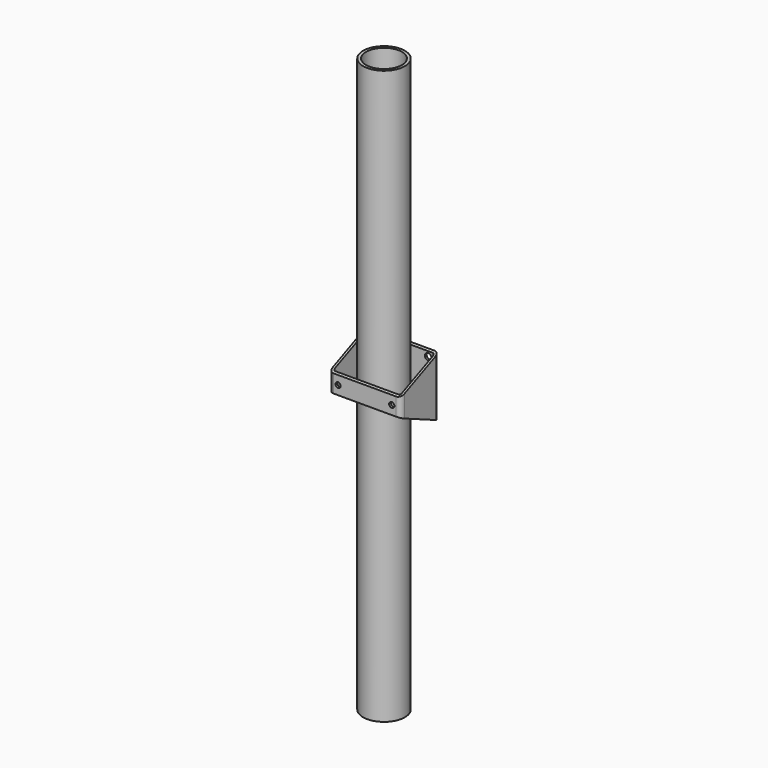
from build123d import *

# Parameters (mm, degrees)
F5_REACH        = 246.7313465507
F7_R            = 44.45
F7_R_2          = 38.1000004709
F8_DEPTH        = 609.6
F8_DEPTH_BACK   = 609.6
F10_D           = 14.3002
F11_D           = 11.1125
F11_CSINK_D     = 19.05
F11_CSINK_ANGLE = 90


with BuildPart() as f5:
    f5_end = Plane(origin=(0, 50.6421849132, 63.5), x_dir=(0, 0.9155220939, 0.4022676914), z_dir=(0, -0.4022676914, 0.9155220939))
    # F0 (on Top) → F5 (new body, up to a plane its end follows)
    with BuildSketch(Plane.XY):
        with BuildLine():
            ThreePointArc((76.2, 41.275), (73.4101920908, 48.0101920908), (66.675, 50.8))
            Line((66.675, 50.8), (-66.675, 50.8))
            ThreePointArc((-66.675, 50.8), (-73.4101920908, 48.0101920908), (-76.2, 41.275))
            Line((-76.2, 41.275), (-76.2, -41.275))
            ThreePointArc((-76.2, -41.275), (-73.4101920908, -48.0101920908), (-66.675, -50.8))
            Line((-66.675, -50.8), (66.675, -50.8))
            ThreePointArc((66.675, -50.8), (73.4101920908, -48.0101920908), (76.2, -41.275))
            Line((76.2, -41.275), (76.2, 41.275))
        make_face()
        with BuildLine():
            ThreePointArc((66.675, 46.0375), (70.0425960454, 44.6425960454), (71.4375, 41.275))
            Line((71.4375, 41.275), (71.4375, -41.275))
            ThreePointArc((71.4375, -41.275), (70.0425960454, -44.6425960454), (66.675, -46.0375))
            Line((66.675, -46.0375), (-66.675, -46.0375))
            ThreePointArc((-66.675, -46.0375), (-70.0425960454, -44.6425960454), (-71.4375, -41.275))
            Line((-71.4375, -41.275), (-71.4375, 41.275))
            ThreePointArc((-71.4375, 41.275), (-70.0425960454, 44.6425960454), (-66.675, 46.0375))
            Line((-66.675, 46.0375), (66.675, 46.0375))
        make_face(mode=Mode.SUBTRACT)
    f5_long = extrude(amount=F5_REACH, mode=Mode.PRIVATE)
    add(split(f5_long, bisect_by=f5_end, keep=Keep.BOTTOM, mode=Mode.PRIVATE))

    # F6: F5 across plane


with BuildPart() as f5_1:
    add(f5.part)
    add(f5.part.mirror(Plane.XY))

    # F10 (through all)
    with Locations(Plane(origin=(0, 50.8, 0), x_dir=(-1, 0, 0), z_dir=(0, 1, 0))):
        with Locations((-57.15, 50.8), (57.15, 50.8), (57.15, -50.8), (-57.15, -50.8)):
            Hole(F10_D / 2)

    # F11 (through all)
    with Locations(Plane(origin=(0, 50.8, 0), x_dir=(-1, 0, 0), z_dir=(0, 1, 0))):
        with Locations((-57.15, 0), (57.15, 0)):
            CounterSinkHole(F11_D / 2, F11_CSINK_D / 2, counter_sink_angle=F11_CSINK_ANGLE)


with BuildPart() as f8:
    # F7 (on Top) → F8 (new body, two sides)
    with BuildSketch(Plane.XY) as f8_sk:
        Circle(F7_R)
        Circle(F7_R_2, mode=Mode.SUBTRACT)
    extrude(amount=F8_DEPTH)
    extrude(f8_sk.sketch, amount=-F8_DEPTH_BACK)


solid = Compound([f5_1.part, f8.part])
